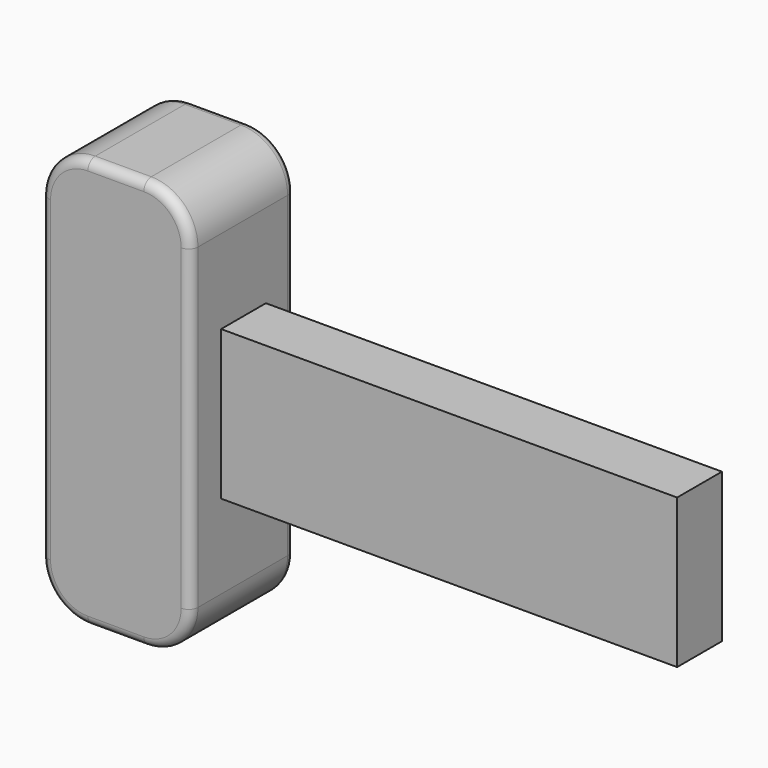
from build123d import *

# Parameters (mm, degrees)
F1_DEPTH = 44.45
F2_R     = 3.175
F3_W     = 19.05
F3_H     = 50.8
F4_DEPTH = 155.1632549


# Not quite as in the source:
# - an extrude ends at something that could not be found from the text; its depth is read off the source's solid


with BuildPart() as f1:
    # F0 (on Front) → F1 (new body)
    with BuildSketch(Plane.XZ):
        with BuildLine():
            Line((9.525, 69.85), (-9.525, 69.85))
            ThreePointArc((-9.525, 69.85), (-20.7503201513, 65.2003201513), (-25.4, 53.975))
            Line((-25.4, 53.975), (-25.4, -53.975))
            ThreePointArc((-25.4, -53.975), (-20.7503201513, -65.2003201513), (-9.525, -69.85))
            Line((-9.525, -69.85), (9.525, -69.85))
            ThreePointArc((9.525, -69.85), (20.7503201513, -65.2003201513), (25.4, -53.975))
            Line((25.4, -53.975), (25.4, 53.975))
            ThreePointArc((25.4, 53.975), (20.7503201513, 65.2003201513), (9.525, 69.85))
        make_face()
    extrude(amount=F1_DEPTH)

    # F2
    f2_edges = [f1.edges().sort_by_distance(p)[0] for p in [
        (0, -44.45, 69.85),
        (20.75032, 0, 65.20032),
        (0, 0, 69.85),
        (-20.75032, 0, 65.20032),
        (-20.75032, -44.45, 65.20032),
        (-25.4, 0, 0),
        (-25.4, -44.45, 0),
        (-20.75032, 0, -65.20032),
        (-20.75032, -44.45, -65.20032),
        (0, 0, -69.85),
        (0, -44.45, -69.85),
        (20.75032, 0, -65.20032),
        (20.75032, -44.45, -65.20032),
        (25.4, 0, 0),
        (25.4, -44.45, 0),
        (20.75032, -44.45, 65.20032),
    ]]
    fillet(f2_edges, radius=F2_R)

    # F3 (on face) → F4 (join, through all)
    with BuildSketch(Plane.YZ.offset(25.4)):
        with Locations((-21.9233557582, 0)):
            Rectangle(F3_W, F3_H)
    extrude(amount=F4_DEPTH)


solid = f1.part
